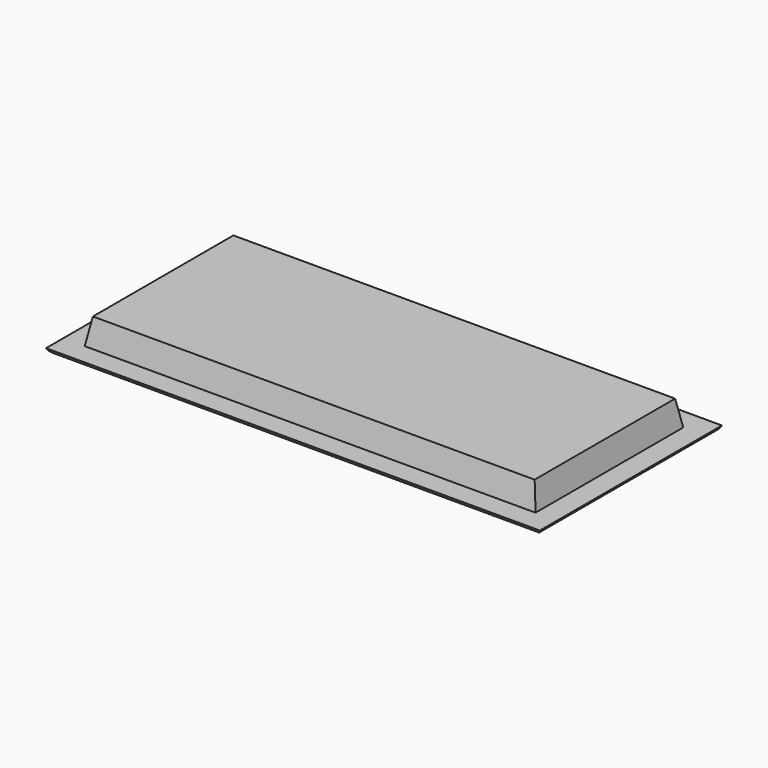
from build123d import *

# Parameters (mm, degrees)
F0_W         = 210
F0_H         = 86
F1_DEPTH     = 15
F0_W_2       = 230
F0_H_2       = 106
F2_DEPTH     = 3
F3_T1_DEPTH  = 252.9128784748
F3_T3_DEPTH  = 128.9128784748
F4_T4_DEPTH  = 272.3649311141
F4_T9_DEPTH  = 148.3649311141
F4_T14_DEPTH = 272.3649311141
F4_T19_DEPTH = 148.3649311141


# Not quite as in the source:
# - a fillet or chamfer that OpenCascade refuses, or shapes differently, is made with other operations: its cross-section is extruded or revolved along the edge and cut away or added


with BuildPart() as f1:
    # F0 (on Top) → F1 (new body)
    with BuildSketch(Plane.XY):
        Rectangle(F0_W, F0_H)
    extrude(amount=F1_DEPTH)

    # F0 (on Top) → F2 (join)
    with BuildSketch(Plane.XY):
        Rectangle(F0_W_2, F0_H_2)
        Rectangle(F0_W, F0_H, mode=Mode.SUBTRACT)
    extrude(amount=F2_DEPTH)

    # F3: fillet of radius 5 on 4 edges, made by hand

    # F3_s2 → F3_t1 (cut)
    with BuildSketch(Plane.YZ.offset(-126.4564392374)):
        with BuildLine():
            ThreePointArc((-53, 3), (-51.1560370926, 0.8166998673), (-48.417424305, 0))
            Line((-48.417424305, 0), (-53, 0))
            Line((-53, 0), (-53, 3))
        make_face()
        with BuildLine():
            ThreePointArc((53, 3), (51.1560370926, 0.8166998673), (48.417424305, 0))
            Line((48.417424305, 0), (53, 0))
            Line((53, 0), (53, 3))
        make_face()
    extrude(amount=F3_T1_DEPTH, mode=Mode.SUBTRACT)

    # F3_s4 → F3_t3 (cut)
    with BuildSketch(Plane.XZ.offset(-64.4564392374)):
        with BuildLine():
            ThreePointArc((115, 3), (113.1560370926, 0.8166998673), (110.417424305, 0))
            Line((110.417424305, 0), (115, 0))
            Line((115, 0), (115, 3))
        make_face()
        with BuildLine():
            ThreePointArc((-115, 3), (-113.1560370926, 0.8166998673), (-110.417424305, 0))
            Line((-110.417424305, 0), (-115, 0))
            Line((-115, 0), (-115, 3))
        make_face()
    extrude(amount=F3_T3_DEPTH, mode=Mode.SUBTRACT)

    # F4: chamfer of 12 x 2.1159237685 on 4 edges, made by hand


with BuildPart() as f4_tool2:
    # F4_s3 → F4_t4 (new body)
    with BuildSketch(Plane.YZ.offset(-136.1824655571)):
        Polygon((-43, 3), (-40.8840762315, 15), (-43, 15), align=None)
    extrude(amount=F4_T4_DEPTH)

    split(bisect_by=Plane.XY.offset(3), keep=Keep.TOP)


with BuildPart() as f1_1:
    add(f1.part)

    # F4_t1: cut F4_tool2
    add(f4_tool2.part, mode=Mode.SUBTRACT)


with BuildPart() as f4_tool7:
    # F4_s8 → F4_t9 (new body)
    with BuildSketch(Plane.XZ.offset(74.1824655571)):
        Polygon((105, 3), (102.8840762315, 15), (105, 15), align=None)
    extrude(amount=-F4_T9_DEPTH)

    split(bisect_by=Plane.XY.offset(3), keep=Keep.TOP)


with BuildPart() as f1_2:
    add(f1_1.part)

    # F4_t6: cut F4_tool7
    add(f4_tool7.part, mode=Mode.SUBTRACT)


with BuildPart() as f4_tool12:
    # F4_s13 → F4_t14 (new body)
    with BuildSketch(Plane.YZ.offset(136.1824655571)):
        Polygon((40.8840762315, 15), (43, 3), (43, 15), align=None)
    extrude(amount=-F4_T14_DEPTH)

    split(bisect_by=Plane.XY.offset(3), keep=Keep.TOP)


with BuildPart() as f1_3:
    add(f1_2.part)

    # F4_t11: cut F4_tool12
    add(f4_tool12.part, mode=Mode.SUBTRACT)


with BuildPart() as f4_tool17:
    # F4_s18 → F4_t19 (new body)
    with BuildSketch(Plane.XZ.offset(-74.1824655571)):
        Polygon((-102.8840762315, 15), (-105, 3), (-105, 15), align=None)
    extrude(amount=F4_T19_DEPTH)

    split(bisect_by=Plane.XY.offset(3), keep=Keep.TOP)


with BuildPart() as f1_4:
    add(f1_3.part)

    # F4_t16: cut F4_tool17
    add(f4_tool17.part, mode=Mode.SUBTRACT)


solid = f1_4.part
